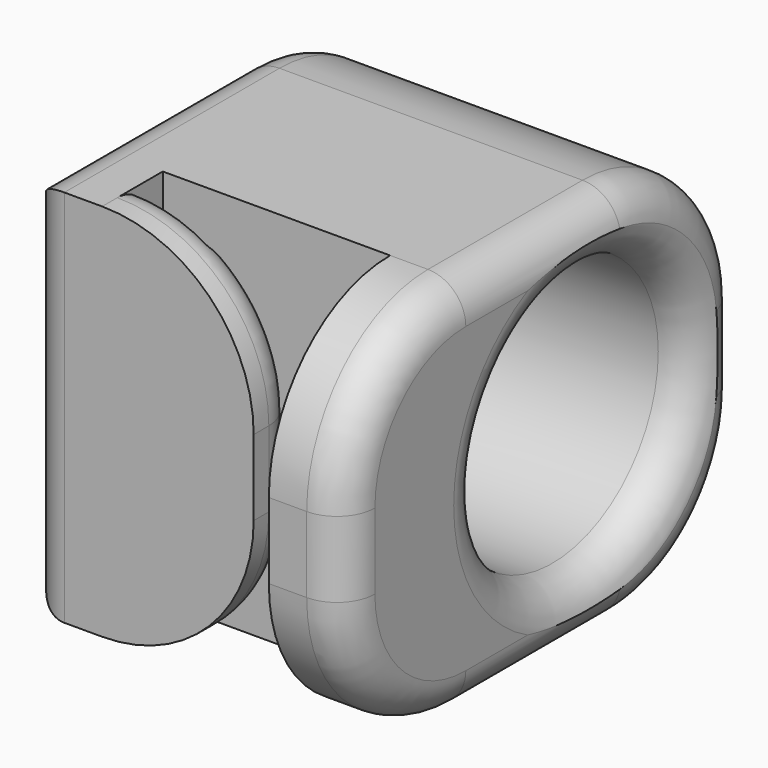
from build123d import *

# Parameters (mm, degrees)
F1_DEPTH     = 5
F2_R         = 3.5
F3_DEPTH     = 12.5
F4_R         = 4
F5_T1_DEPTH  = 9.6
F5_T3_DEPTH  = 2
F5_T5_DEPTH  = 15
F5_T7_DEPTH  = 5.1
F5_T9_DEPTH  = 13.2583302492
F5_T12_ANGLE = 90
F5_T14_ANGLE = 90
F5_T18_ANGLE = 90
F5_T20_ANGLE = 90
F5_T22_ANGLE = 90
F5_T24_ANGLE = 90
F5_T30_ANGLE = 95.816254581
F5_T35_ANGLE = 95.816254581


# Not quite as in the source:
# - a fillet or chamfer that OpenCascade refuses, or shapes differently, is made with other operations: its cross-section is extruded or revolved along the edge and cut away or added


with BuildPart() as f1:
    # F0 (on Top) → F1 (new body, symmetric)
    with BuildSketch(Plane.XY):
        Polygon((2, -2), (2, -1), (5, -1), (8, -1), (8, -5), (10, -5), (10, 0), (10, 8.1), (0, 8.1), (0, 0), (0, -3), (6, -3), (6, -1.5), (4, -1.5), (4, -2), align=None)
    extrude(amount=F1_DEPTH, both=True)

    # F2 (on face) → F3 (cut, symmetric)
    with BuildSketch(Plane.YZ.offset(10)):
        with Locations((3.1, 0)):
            Circle(F2_R)
    extrude(amount=F3_DEPTH, both=True, mode=Mode.SUBTRACT)

    # F4
    f4_edges = [f1.edges().sort_by_distance(p)[0] for p in [
        (5, 8.1, -5),
        (5, 8.1, 5),
        (9, -5, -5),
        (9, -5, 5),
        (6, -2.25, 5),
        (6, -2.25, -5),
    ]]
    fillet(f4_edges, radius=F4_R)

    # F5: fillet of radius 1 on 20 edges, made by hand

    # F5_s2 → F5_t1 (cut)
    with BuildSketch(Plane.XZ.offset(-4.1)):
        with BuildLine():
            ThreePointArc((0, 4), (0.2928932188, 4.7071067812), (1, 5))
            Line((1, 5), (0, 5))
            Line((0, 5), (0, 4))
        make_face()
        with BuildLine():
            ThreePointArc((1, -5), (0.2928932188, -4.7071067812), (0, -4))
            Line((0, -4), (0, -5))
            Line((0, -5), (1, -5))
        make_face()
    extrude(amount=F5_T1_DEPTH, mode=Mode.SUBTRACT)

    # F5_s4 → F5_t3 (cut)
    with BuildSketch(Plane.XY.offset(-1)):
        with BuildLine():
            ThreePointArc((0, 7.1), (0.2928932188, 7.8071067812), (1, 8.1))
            Line((1, 8.1), (0, 8.1))
            Line((0, 8.1), (0, 7.1))
        make_face()
        with BuildLine():
            ThreePointArc((10, -4), (9.7071067812, -4.7071067812), (9, -5))
            Line((9, -5), (10, -5))
            Line((10, -5), (10, -4))
        make_face()
        with BuildLine():
            ThreePointArc((10, 7.1), (9.7071067812, 7.8071067812), (9, 8.1))
            Line((9, 8.1), (10, 8.1))
            Line((10, 8.1), (10, 7.1))
        make_face()
        with BuildLine():
            ThreePointArc((6, -2.5), (5.7071067812, -1.7928932188), (5, -1.5))
            Line((5, -1.5), (6, -1.5))
            Line((6, -1.5), (6, -2.5))
        make_face()
    extrude(amount=F5_T3_DEPTH, mode=Mode.SUBTRACT)

    # F5_s6 → F5_t5 (cut)
    with BuildSketch(Plane.XY.offset(-7.5)):
        with BuildLine():
            ThreePointArc((0, -2), (0.2928932188, -2.7071067812), (1, -3))
            Line((1, -3), (0, -3))
            Line((0, -3), (0, -2))
        make_face()
    extrude(amount=F5_T5_DEPTH, mode=Mode.SUBTRACT)

    # F5_s8 → F5_t7 (cut)
    with BuildSketch(Plane.XZ.offset(-4.1)):
        with BuildLine():
            ThreePointArc((9, -5), (9.7071067812, -4.7071067812), (10, -4))
            Line((10, -4), (10, -5))
            Line((10, -5), (9, -5))
        make_face()
        with BuildLine():
            ThreePointArc((10, 4), (9.7071067812, 4.7071067812), (9, 5))
            Line((9, 5), (10, 5))
            Line((10, 5), (10, 4))
        make_face()
    extrude(amount=F5_T7_DEPTH, mode=Mode.SUBTRACT)

    # F5_s10 → F5_t9 (cut)
    with BuildSketch(Plane.XY.offset(-6.6291651246)):
        with BuildLine():
            ThreePointArc((4, -2), (4.3660254038, -1.6339745962), (4.8660254038, -1.5))
            Line((4.8660254038, -1.5), (4, -1.5))
            Line((4, -1.5), (4, -2))
        make_face()
    extrude(amount=F5_T9_DEPTH, mode=Mode.SUBTRACT)

    # F5_s11 → F5_t12 (revolve, cut)
    with BuildSketch(Plane.XZ.offset(-4.1)):
        with BuildLine():
            ThreePointArc((1, -5), (0.2928932188, -4.7071067812), (0, -4))
            Line((0, -4), (0, -5))
            Line((0, -5), (1, -5))
        make_face()
    revolve(axis=Axis((0, 4.1, -1), (1, 0, 0)), revolution_arc=F5_T12_ANGLE, mode=Mode.SUBTRACT)

    # F5_s13 → F5_t14 (revolve, cut)
    with BuildSketch(Plane.XZ.offset(-4.1)):
        with BuildLine():
            ThreePointArc((0, 4), (0.2928932188, 4.7071067812), (1, 5))
            Line((1, 5), (0, 5))
            Line((0, 5), (0, 4))
        make_face()
    revolve(axis=Axis((0, 4.1, 1), (-1, 0, 0)), revolution_arc=F5_T14_ANGLE, mode=Mode.SUBTRACT)

    # F5_s15 → F5_t16 (revolve, cut)
    with BuildSketch(Plane.XY):
        with BuildLine():
            ThreePointArc((0, 7.6), (0.2928932188, 6.8928932188), (1, 6.6))
            Line((1, 6.6), (0, 6.6))
            Line((0, 6.6), (0, 7.6))
        make_face()
    revolve(axis=Axis((0, 3.1, 0), (1, 0, 0)), mode=Mode.SUBTRACT)

    # F5_s17 → F5_t18 (revolve, cut)
    with BuildSketch(Plane.XZ.offset(1)):
        with BuildLine():
            ThreePointArc((10, -4), (9.7071067812, -4.7071067812), (9, -5))
            Line((9, -5), (10, -5))
            Line((10, -5), (10, -4))
        make_face()
    revolve(axis=Axis((10, -1, -1), (-1, 0, 0)), revolution_arc=F5_T18_ANGLE, mode=Mode.SUBTRACT)

    # F5_s19 → F5_t20 (revolve, cut)
    with BuildSketch(Plane.XZ.offset(1)):
        with BuildLine():
            ThreePointArc((10, 4), (9.7071067812, 4.7071067812), (9, 5))
            Line((9, 5), (10, 5))
            Line((10, 5), (10, 4))
        make_face()
    revolve(axis=Axis((10, -1, 1), (1, 0, 0)), revolution_arc=F5_T20_ANGLE, mode=Mode.SUBTRACT)

    # F5_s21 → F5_t22 (revolve, cut)
    with BuildSketch(Plane.XZ.offset(-4.1)):
        with BuildLine():
            ThreePointArc((10, -4), (9.7071067812, -4.7071067812), (9, -5))
            Line((9, -5), (10, -5))
            Line((10, -5), (10, -4))
        make_face()
    revolve(axis=Axis((10, 4.1, -1), (1, 0, 0)), revolution_arc=F5_T22_ANGLE, mode=Mode.SUBTRACT)

    # F5_s23 → F5_t24 (revolve, cut)
    with BuildSketch(Plane.XZ.offset(-4.1)):
        with BuildLine():
            ThreePointArc((10, 4), (9.7071067812, 4.7071067812), (9, 5))
            Line((9, 5), (10, 5))
            Line((10, 5), (10, 4))
        make_face()
    revolve(axis=Axis((10, 4.1, 1), (-1, 0, 0)), revolution_arc=F5_T24_ANGLE, mode=Mode.SUBTRACT)

    # F5_s25 → F5_t26 (revolve, cut)
    with BuildSketch(Plane.XY):
        with BuildLine():
            ThreePointArc((10, 7.6), (9.7071067812, 6.8928932188), (9, 6.6))
            Line((9, 6.6), (10, 6.6))
            Line((10, 6.6), (10, 7.6))
        make_face()
    revolve(axis=Axis((10, 3.1, 0), (1, 0, 0)), mode=Mode.SUBTRACT)


with BuildPart() as f5_tool28:
    # F5_s29 → F5_t30 (revolve)
    with BuildSketch(Plane(origin=(2.0802778479, 0, -0.2119031909), x_dir=(0, 1, 0), z_dir=(-0.9948519995, 0, 0.1013385367))):
        with BuildLine():
            ThreePointArc((-2.5, 4.792174926), (-1.7928932188, 4.4992817072), (-1.5, 3.792174926))
            Line((-1.5, 3.792174926), (-1.5, 4.792174926))
            Line((-1.5, 4.792174926), (-2.5, 4.792174926))
        make_face()
    revolve(axis=Axis((2, -1.5, -1), (0, -1, 0)), revolution_arc=F5_T30_ANGLE)

    split(bisect_by=Plane.YZ.offset(2), keep=Keep.TOP)


with BuildPart() as f1_1:
    add(f1.part)

    # F5_t27: cut F5_tool28
    add(f5_tool28.part, mode=Mode.SUBTRACT)


with BuildPart() as f5_tool33:
    # F5_s34 → F5_t35 (revolve)
    with BuildSketch(Plane(origin=(2.0802778479, 0, 0.2119031909), x_dir=(0, 1, 0), z_dir=(-0.9948519995, 0, -0.1013385367))):
        with BuildLine():
            ThreePointArc((-2.5, -4.792174926), (-1.7928932188, -4.4992817072), (-1.5, -3.792174926))
            Line((-1.5, -3.792174926), (-1.5, -4.792174926))
            Line((-1.5, -4.792174926), (-2.5, -4.792174926))
        make_face()
    revolve(axis=Axis((2, -1.5, 1), (0, 1, 0)), revolution_arc=F5_T35_ANGLE)

    split(bisect_by=Plane.YZ.offset(2), keep=Keep.TOP)


with BuildPart() as f1_2:
    add(f1_1.part)

    # F5_t32: cut F5_tool33
    add(f5_tool33.part, mode=Mode.SUBTRACT)


solid = f1_2.part
